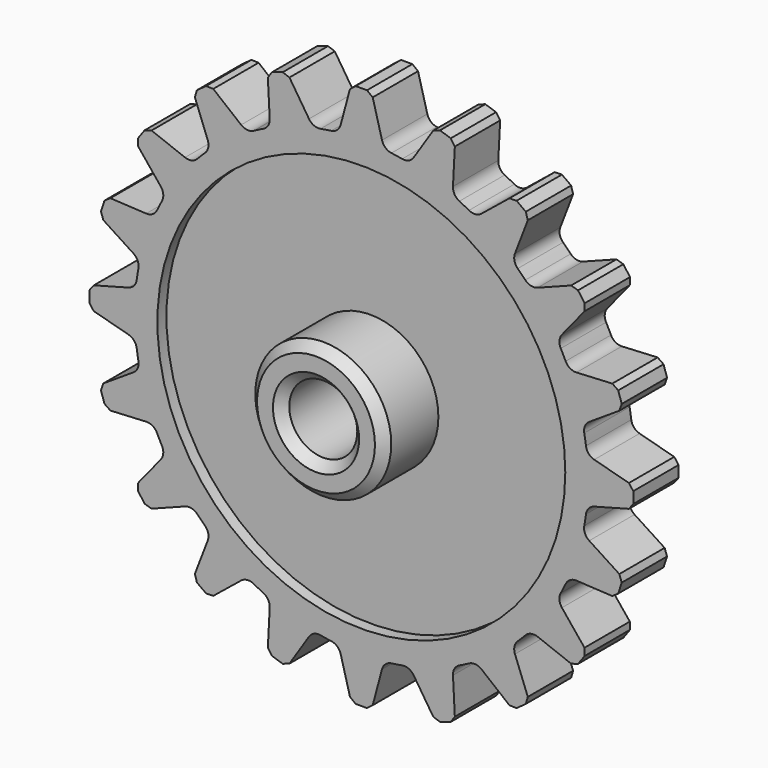
from build123d import *

# Parameters (mm, degrees)
F0_R            = 100
F1_DEPTH        = 25
F3_DEPTH        = 25
F3_COPIES_COUNT = 20
F4_R            = 5
F5_SIZE         = 2
F6_R            = 90
F7_DEPTH        = 5
F8_R            = 30
F9_DEPTH        = 30
F10_R           = 15
F11_DEPTH       = 50.001
F12_SIZE        = 4


# Not quite as in the source:
# - a pattern or mirror of a feature is missing from the dataset's text; its kind, count and spacing are read off the source's solid


with BuildPart() as f1:
    # F0 (on Front) → F1 (new body)
    with BuildSketch(Plane.XZ):
        Circle(F0_R)
    extrude(amount=F1_DEPTH)

    # F2 (on face) → F3 (join)
    with BuildSketch(Plane.XZ.offset(25)):
        Polygon((-4.5, 120), (-9.9931095726, 99.4994359837), (9.9931095726, 99.4994359837), (4.5, 120), align=None)
    f3 = extrude(amount=-F3_DEPTH)

    # F3_copies: F3 ×20 about axis
    f3_copies_axis = Axis((0, 0, 0), (0, 1, 0))
    for i in range(1, F3_COPIES_COUNT):
        add(f3.rotate(f3_copies_axis, i * 360 / F3_COPIES_COUNT))

    # F4
    f4_edges = [f1.edges().sort_by_distance(p)[0] for p in [
        (9.99311, -12.5, 99.499436),
        (-9.99311, -12.5, 99.499436),
        (-21.243005, -12.5, 97.717628),
        (97.717628, -12.5, 21.243005),
        (99.499436, -12.5, 9.99311),
        (99.499436, -12.5, -9.99311),
        (97.717628, -12.5, -21.243005),
        (91.541546, -12.5, -40.251029),
        (86.370537, -12.5, -50.399706),
        (74.622932, -12.5, -66.568897),
        (66.568897, -12.5, -74.622932),
        (50.399706, -12.5, -86.370537),
        (40.251029, -12.5, -91.541546),
        (21.243005, -12.5, -97.717628),
        (9.99311, -12.5, -99.499436),
        (-9.99311, -12.5, -99.499436),
        (-21.243005, -12.5, -97.717628),
        (-40.251029, -12.5, -91.541546),
        (-50.399706, -12.5, -86.370537),
        (-66.568897, -12.5, -74.622932),
        (-74.622932, -12.5, -66.568897),
        (-86.370537, -12.5, -50.399706),
        (-91.541546, -12.5, -40.251029),
        (-97.717628, -12.5, -21.243005),
        (-99.499436, -12.5, -9.99311),
        (-99.499436, -12.5, 9.99311),
        (-97.717628, -12.5, 21.243005),
        (-91.541546, -12.5, 40.251029),
        (-86.370537, -12.5, 50.399706),
        (-74.622932, -12.5, 66.568897),
        (-66.568897, -12.5, 74.622932),
        (-50.399706, -12.5, 86.370537),
        (-40.251029, -12.5, 91.541546),
        (21.243005, -12.5, 97.717628),
        (40.251029, -12.5, 91.541546),
        (50.399706, -12.5, 86.370537),
        (66.568897, -12.5, 74.622932),
        (74.622932, -12.5, 66.568897),
        (86.370537, -12.5, 50.399706),
        (91.541546, -12.5, 40.251029),
    ]]
    fillet(f4_edges, radius=F4_R)

    # F5
    f5_edges = [f1.edges().sort_by_distance(p)[0] for p in [
        (-4.5, -12.5, 120),
        (4.5, -12.5, 120),
        (115.517358, -12.5, 32.802285),
        (112.736205, -12.5, 41.361794),
        (120, -12.5, 4.5),
        (120, -12.5, -4.5),
        (99.727073, -12.5, 66.893654),
        (94.437006, -12.5, 74.174807),
        (115.517358, -12.5, -32.802285),
        (112.736205, -12.5, -41.361794),
        (74.174807, -12.5, 94.437006),
        (66.893654, -12.5, 99.727073),
        (99.727073, -12.5, -66.893654),
        (94.437006, -12.5, -74.174807),
        (41.361794, -12.5, 112.736205),
        (32.802285, -12.5, 115.517358),
        (74.174807, -12.5, -94.437006),
        (66.893654, -12.5, -99.727073),
        (41.361794, -12.5, -112.736205),
        (32.802285, -12.5, -115.517358),
        (-32.802285, -12.5, 115.517358),
        (-41.361794, -12.5, 112.736205),
        (4.5, -12.5, -120),
        (-4.5, -12.5, -120),
        (-66.893654, -12.5, 99.727073),
        (-74.174807, -12.5, 94.437006),
        (-32.802285, -12.5, -115.517358),
        (-41.361794, -12.5, -112.736205),
        (-94.437006, -12.5, 74.174807),
        (-99.727073, -12.5, 66.893654),
        (-66.893654, -12.5, -99.727073),
        (-74.174807, -12.5, -94.437006),
        (-112.736205, -12.5, 41.361794),
        (-115.517358, -12.5, 32.802285),
        (-94.437006, -12.5, -74.174807),
        (-99.727073, -12.5, -66.893654),
        (-120, -12.5, 4.5),
        (-120, -12.5, -4.5),
        (-112.736205, -12.5, -41.361794),
        (-115.517358, -12.5, -32.802285),
    ]]
    chamfer(f5_edges, length=F5_SIZE)

    # F6 (on face) → F7 (cut)
    with BuildSketch(Plane.XZ.offset(25)):
        Circle(F6_R)
    extrude(amount=-F7_DEPTH, mode=Mode.SUBTRACT)

    # F8 (on face) → F9 (join)
    with BuildSketch(Plane.XZ.offset(20)):
        Circle(F8_R)
    extrude(amount=F9_DEPTH)

    # F10 (on face) → F11 (cut, through all)
    with BuildSketch(Plane.XZ.offset(50)):
        Circle(F10_R)
    extrude(amount=-F11_DEPTH, mode=Mode.SUBTRACT)

    # F12
    f12_edges = [f1.edges().sort_by_distance(p)[0] for p in [
        (-30, -50, 0),
        (-15, -50, 0),
    ]]
    chamfer(f12_edges, length=F12_SIZE)


solid = f1.part
